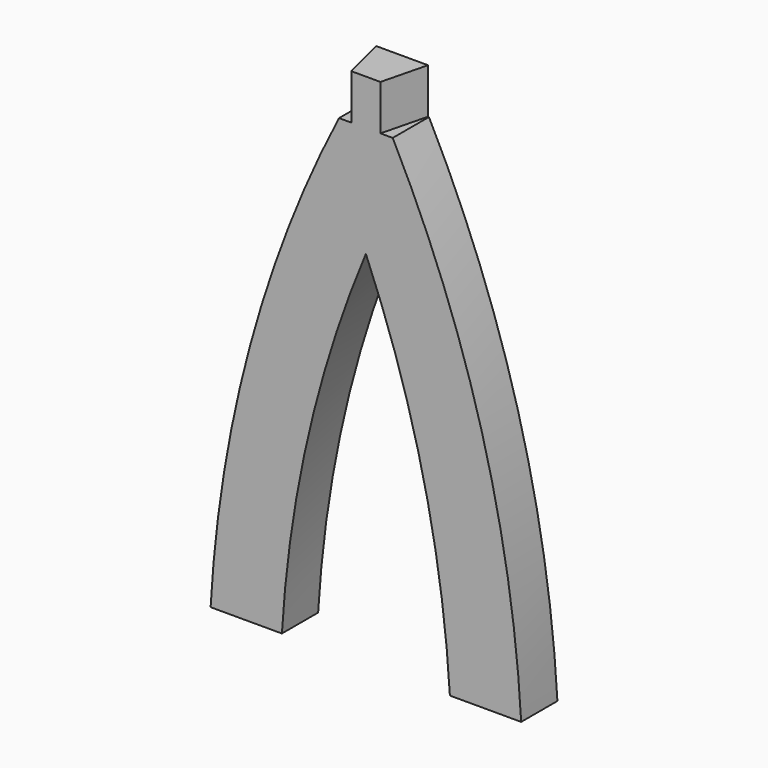
from build123d import *

# Parameters (mm, degrees)
F2_DEPTH = 88.9
F3_W     = 26.7864570916
F3_H     = 88.9
F4_DEPTH = 88.9


# Not quite as in the source:
# - a variable given as a bare number and used for a length is read in inches; the dataset says mm whatever the document's units were


with BuildPart() as f2:
    # F1 (on Front) → F2 (new body)
    with BuildSketch(Plane.XZ):
        with BuildLine():
            Line((85.6085425377, 530.4986528046), (34.8085425377, 530.4986528046))
            Line((34.8085425377, 530.4986528046), (-15.9914574623, 530.4986528046))
            Line((-15.9914574623, 530.4986528046), (-17.8685326312, 441.5986528046))
            ThreePointArc((-17.8685326312, 441.5986528046), (-192.6665275597, -8.6975481194), (-269.9914574623, -485.5013471954))
            Line((-269.9914574623, -485.5013471954), (-130.0577898718, -485.5013471954))
            ThreePointArc((-130.0577898718, -485.5013471954), (-77.615001681, -123.7260262863), (34.8085425377, 224.1138442826))
            ThreePointArc((34.8085425377, 224.1138442826), (147.2320867564, -123.7260262863), (199.6748749472, -485.5013471954))
            Line((199.6748749472, -485.5013471954), (339.6085425377, -485.5013471954))
            ThreePointArc((339.6085425377, -485.5013471954), (262.2836126351, -8.6975481194), (87.4856177066, 441.5986528046))
            Line((87.4856177066, 441.5986528046), (85.6085425377, 530.4986528046))
        make_face()
    extrude(amount=F2_DEPTH)

    # F3 (on face) → F4 (cut)
    with BuildSketch(Plane.XY.offset(530.4986528046)):
        Polygon((-15.9914574623, -88.9), (6.2335425377, -88.9), (-15.9914574623, 0), align=None)
        Polygon((85.6085425377, 0), (63.3835425377, -88.9), (85.6085425377, -88.9), align=None)
        Polygon((122.7087825537, 0), (85.6085425377, 0), (85.6085425377, -88.9), (129.0911585093, -88.9), align=None)
        with Locations((-29.3846860081, -44.45)):
            Rectangle(F3_W, F3_H)
    extrude(amount=-F4_DEPTH, mode=Mode.SUBTRACT)


solid = f2.part
